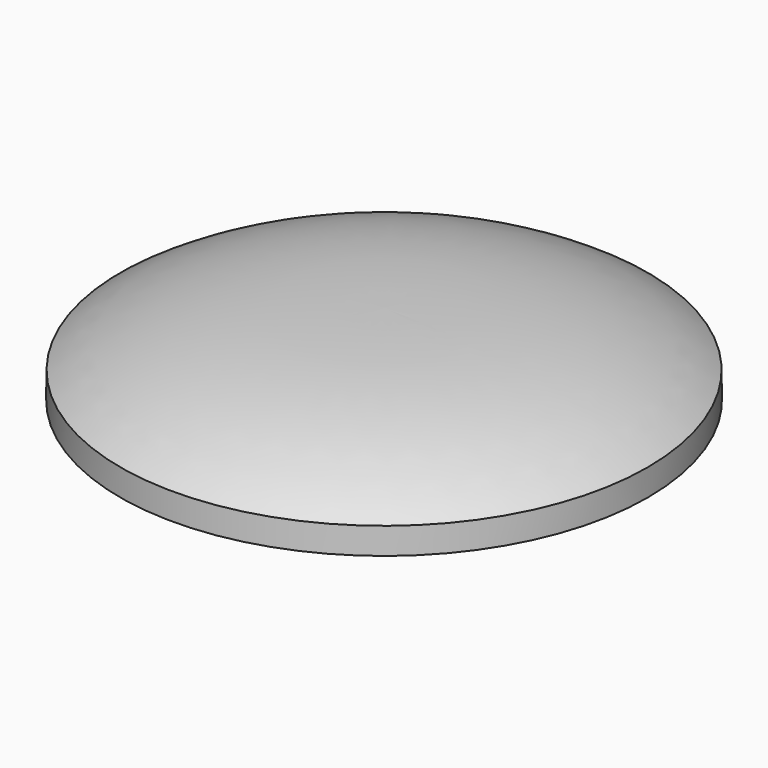
from build123d import *

# Parameters (mm, degrees)
F3_TEXT_SIZE   = 3.7933534865
F3_TEXT_SIZE_2 = 5.585638347
F4_DEPTH       = 0.05


# Not quite as in the source:
# - Text() gives the source's letters only with a copy of the font that has no kerning and outlines rounded to 1/6400 em; it was checked with that copy


with BuildPart() as f1:
    # F0 (on Front) → F1 (revolve)
    with BuildSketch(Plane.XZ):
        with BuildLine():
            Line((0, 3.0717726331), (0, 0))
            Line((0, 0), (10.0135328248, 0))
            Line((10.0135328248, 0), (10, 1))
            add(Edge.make_bspline(
                [(10, 1), (6.9053554907, 3.1140228966), (2.5164748076, 3.0511349905), (0, 3.0717726331)],
                knots=[0, 0, 0, 0, 10.2123573108, 10.2123573108, 10.2123573108, 10.2123573108], degree=3))
        make_face()
    revolve(axis=Axis((0, 0, 1.5358863166), (0, 0, 1)))

    # F3 (on offset) → F4 (cut)
    with BuildSketch(Plane.XY.offset(1)):
        with Locations((1.4295794535, 2.6564311702)):
            Text('A', F3_TEXT_SIZE, font='Open Sans', font_style=FontStyle.BOLD, text_align=(TextAlign.LEFT, TextAlign.BOTTOM))
        with Locations((-4.6238657087, -5.7970392518)):
            Text('*', F3_TEXT_SIZE_2, font='Open Sans', font_style=FontStyle.BOLD, text_align=(TextAlign.LEFT, TextAlign.BOTTOM))
    extrude(amount=-F4_DEPTH, mode=Mode.SUBTRACT)


solid = f1.part
